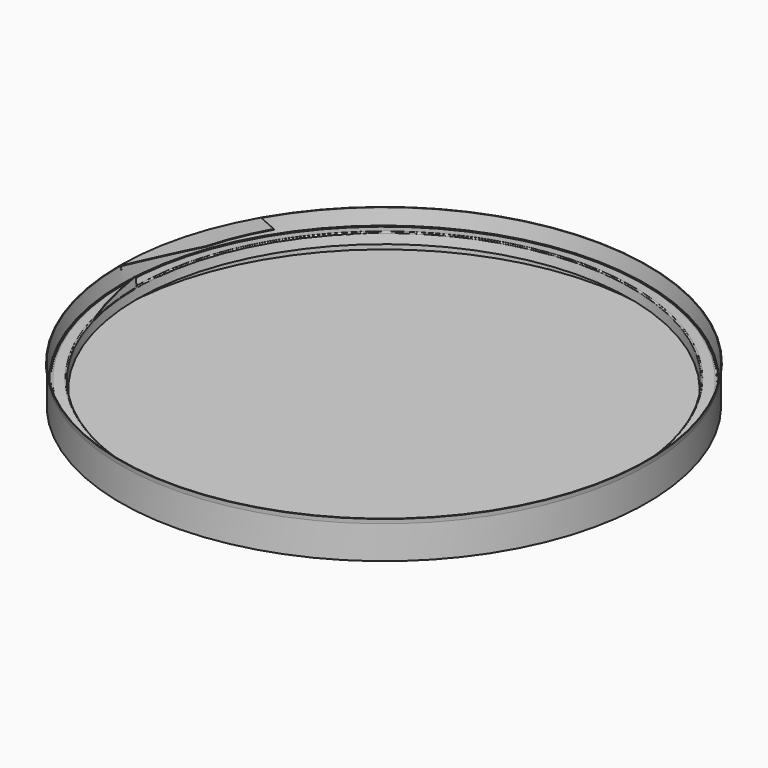
from build123d import *
from build123d import SkipClean  # not in build123d's __all__

# Parameters (mm, degrees)
F4_ANGLE  = 30
F5_R      = 2.54
F8_DEPTH  = 25.4
F9_ANGLE  = 15
F11_DEPTH = 584.2


with BuildPart() as f2:
    # F0 (on Front) → F2 (revolve)
    with BuildSketch(Plane.XZ):
        Polygon((-609.6, 22.2812721531), (-609.6, -3.1187278469), (-609.6, -53.9187278469), (0, -53.9187278469), (0, -52.6487278469), (-608.33, -52.6487278469), (-608.33, -5.9370508356), (-575.9571166824, -1.9621605723), (-573.4033445914, -22.7609651799), (-570.8495725003, -22.4474013951), (-573.4033445914, -1.6485967874), (-573.7902797567, 1.502737244), (-585.1143879206, 0.1123115955), (-598.7488452858, -1.5617892652), (-598.5940712197, -2.8223228778), (-602.3756720575, -3.2866450762), (-602.5304461236, -2.0261114636), (-605.3036200713, -2.3666144091), (-608.33, 22.2812721531), (-609.4515650434, 31.4156864082), (-609.6264646317, 32.840129245), (-610.8776024179, 32.6865088413), (-610.7215650434, 31.4156864082), align=None)
    revolve(axis=Axis((0, 0, -10.9399985522), (0, 0, -1)))

    # F0 (on Front) → F4 (revolve)
    with BuildSketch(Plane.XZ):
        Polygon((-546.5997840024, 40.5788325512), (-609.6264646317, 32.840129245), (-609.4515650434, 31.4156864082), (-546.4248844142, 39.1543897144), align=None)
    with SkipClean():  # cleaning this boolean's faces spoils the solid; the shape is the same uncleaned
        revolve(axis=Axis((0, 0, -10.9399985522), (0, 0, -1)), revolution_arc=F4_ANGLE)

    # F5
    f5_edges = [f2.edges().sort_by_distance(p)[0] for p in [
        (573.79028, 0, 1.502737),
    ]]
    fillet(f5_edges, radius=F5_R)

    # F7 (on offset) → F8 (cut)
    with BuildSketch(Plane.XY.offset(23.5512721531)):
        Polygon((-523.0901241302, 151.6724824905), (-609.3410253525, 0), (-542.667388916, -7.2113391943), align=None)
    with SkipClean():  # cleaning this boolean's faces spoils the solid; the shape is the same uncleaned
        extrude(amount=F8_DEPTH, mode=Mode.SUBTRACT)


with BuildPart() as f9:
    # F0 (on Front) → F9 (revolve)
    with BuildSketch(Plane.XZ):
        Polygon((-576.2698686253, 21.6973679888), (-573.7902797567, 1.502737244), (-572.2845961987, 1.502737244), (-574.7865476856, 21.8794968991), align=None)
    revolve(axis=Axis((0, 0, -10.9399985522), (0, 0, 1)), revolution_arc=F9_ANGLE)

    # F10 (on Right) → F11 (cut)
    with BuildSketch(Plane.YZ):
        Polygon((-149.5092064142, 21.9517517835), (-148.5134363174, 1.5399645781), (0.4650368064, 21.9517517835), align=None)
    extrude(amount=-F11_DEPTH, mode=Mode.SUBTRACT)


solid = Compound([f2.part, f9.part])
